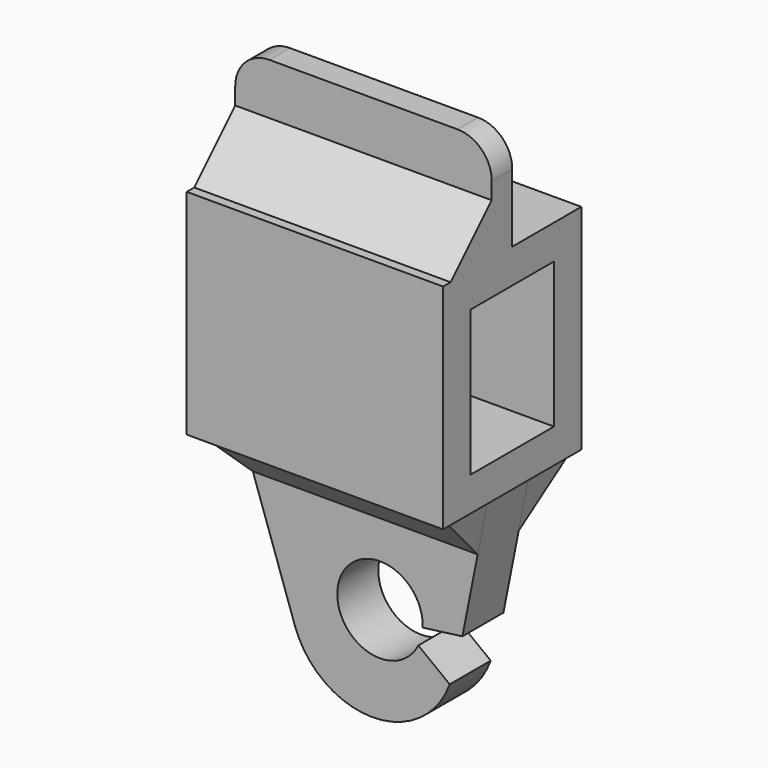
from build123d import *

# Parameters (mm, degrees)
F0_W         = 10.1
F0_H         = 12.5
F0_W_2       = 6.1
F0_H_2       = 8.5
F1_DEPTH     = 15
F3_DEPTH     = 1.5
F5_DEPTH     = 1.5
F6_T1_DEPTH  = 15
F6_T6_DEPTH  = 22.4868112825
F6_T12_DEPTH = 22.4868112825


# Not quite as in the source:
# - a fillet or chamfer that OpenCascade refuses, or shapes differently, is made with other operations: its cross-section is extruded or revolved along the edge and cut away or added


with BuildPart() as f1:
    # F0 (on Right) → F1 (new body)
    with BuildSketch(Plane.YZ):
        Rectangle(F0_W, F0_H)
        Rectangle(F0_W_2, F0_H_2, mode=Mode.SUBTRACT)
    extrude(amount=F1_DEPTH)

    # F2 (on Front) → F3 (join, symmetric)
    with BuildSketch(Plane.XZ):
        with BuildLine():
            Line((14.7717623186, -6.25), (0, -6.25))
            Line((0, -6.25), (3.4864366891, -16.3906378753))
            ThreePointArc((3.4864366891, -16.3906378753), (7.9854016639, -19.6317508441), (12.5416083041, -16.4716115793))
            Line((12.5416083041, -16.4716115793), (10.7079865556, -15.0650723372))
            ThreePointArc((10.7079865556, -15.0650723372), (6.0450329155, -13.3366260518), (10.964385436, -14.0650723372))
            Line((10.964385436, -14.0650723372), (13.2847928678, -13.7592216636))
            Line((13.2847928678, -13.7592216636), (14.7717623186, -6.25))
        make_face()
    extrude(amount=F3_DEPTH, both=True)

    # F4 (on Front) → F5 (join)
    with BuildSketch(Plane.XZ):
        with BuildLine():
            Line((0, 10.25), (0, 6.25))
            Line((0, 6.25), (15, 6.25))
            Line((15, 6.25), (15, 10.25))
            ThreePointArc((15, 10.25), (14.4142135624, 11.6642135624), (13, 12.25))
            Line((13, 12.25), (2, 12.25))
            ThreePointArc((2, 12.25), (0.5857864376, 11.6642135624), (0, 10.25))
        make_face()
    extrude(amount=F5_DEPTH)

    # F6: chamfer of 3 on 3 edges, made by hand

    # F6_s2 → F6_t1 (join)
    with BuildSketch(Plane.YZ):
        Polygon((-4.5, 6.25), (-1.5, 9.25), (-1.5, 6.25), align=None)
    extrude(amount=F6_T1_DEPTH)


with BuildPart() as f6_tool4:
    # F6_s5 → F6_t6 (new body)
    with BuildSketch(Plane.YZ.offset(22.4868112825)):
        Polygon((-4.5, -6.25), (-1.5, -9.25), (-1.5, -6.25), align=None)
    extrude(amount=-F6_T6_DEPTH)

    split(bisect_by=Plane(origin=(15.4053151941, 0, -3.0505469275), x_dir=(0, 1, 0), z_dir=(-0.9809525786, 0, 0.1942473644)), keep=Keep.TOP)

    split(bisect_by=Plane(origin=(-1.9216548906, 0, -0.6606811324), x_dir=(0, 1, 0), z_dir=(0.945669614, 0, 0.3251291761)), keep=Keep.TOP)


with BuildPart() as f1_1:
    add(f1.part)

    # F6_t3: union F6_tool4
    add(f6_tool4.part)


with BuildPart() as f6_tool10:
    # F6_s11 → F6_t12 (new body)
    with BuildSketch(Plane.YZ.offset(22.4868112825)):
        Polygon((4.5, -6.25), (1.5, -9.25), (1.5, -6.25), align=None)
    extrude(amount=-F6_T12_DEPTH)

    split(bisect_by=Plane(origin=(15.4053151941, 0, -3.0505469275), x_dir=(0, 1, 0), z_dir=(-0.9809525786, 0, 0.1942473644)), keep=Keep.TOP)

    split(bisect_by=Plane(origin=(-1.9216548906, 0, -0.6606811324), x_dir=(0, 1, 0), z_dir=(0.945669614, 0, 0.3251291761)), keep=Keep.TOP)


with BuildPart() as f1_2:
    add(f1_1.part)

    # F6_t9: union F6_tool10
    add(f6_tool10.part)


solid = f1_2.part
